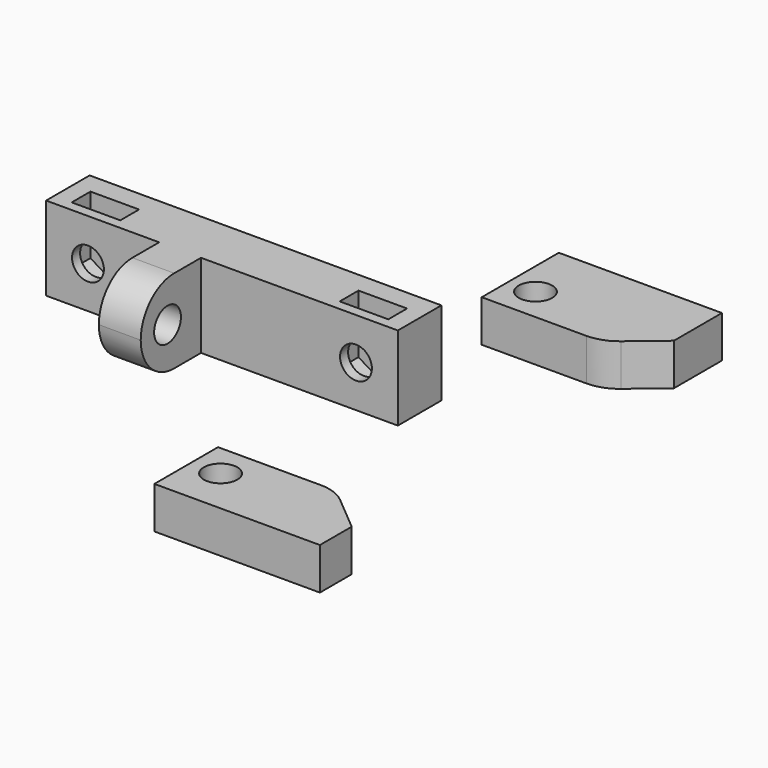
from build123d import *

# Parameters (mm, degrees)
F0_R          = 2
F1_DEPTH      = 5
F2_W          = 5
F2_H          = 9
F3_DEPTH      = 10
F4_R          = 4.99999
F5_R          = 2
F6_DEPTH      = 25
F7_R          = 1.9
F8_DEPTH      = 25
F9_W          = 5.8
F9_H          = 2.8
F10_DEPTH     = 7
F12_DEPTH     = 2.8
F13_TEXT_SIZE = 5.6005794451
F14_DEPTH     = 0.5


# Not quite as in the source:
# - a fillet or chamfer is up to 0.001 mm smaller than in the source, because OpenCascade refuses the exact size
# - Text() gives the source's letters only with a copy of the font that has no kerning and outlines rounded to 1/6400 em; it was checked with that copy


with BuildPart() as f1:
    # F0 (on Top) → F1 (new body)
    with BuildSketch(Plane.XY):
        with BuildLine():
            Line((-19.0093460243, 27.9687746611), (-19.0093460243, 16.4687746611))
            Line((-19.0093460243, 16.4687746611), (-6.5133564216, 16.4687746611))
            ThreePointArc((-6.5133564216, 16.4687746611), (-4.8032557049, 16.7703115571), (-3.2994183731, 17.6385524455))
            Line((-3.2994183731, 17.6385524455), (0.4682703734, 20.8000186831))
            Line((0.4682703734, 20.8000186831), (0.4682703734, 27.9687746611))
            Line((0.4682703734, 27.9687746611), (-19.0093460243, 27.9687746611))
        make_face()
        with Locations((-15.7921736951, 20.4687746611)):
            Circle(F0_R, mode=Mode.SUBTRACT)
    extrude(amount=F1_DEPTH)


with BuildPart() as f1b:
    # F0 (on Top) → F1, piece 2 (new body)
    with BuildSketch(Plane.XY):
        with BuildLine():
            Line((-19.2959401757, -22.5312253389), (-19.2959401757, -32.0312253389))
            Line((-19.2959401757, -32.0312253389), (0.4682703734, -32.0312253389))
            Line((0.4682703734, -32.0312253389), (0.4682703734, -27.2812253389))
            Line((0.4682703734, -27.2812253389), (-3.7984723143, -23.7010031233))
            ThreePointArc((-3.7984723143, -23.7010031233), (-5.3023096461, -22.832762235), (-7.0124103627, -22.5312253389))
            Line((-7.0124103627, -22.5312253389), (-19.2959401757, -22.5312253389))
        make_face()
        with Locations((-15.7921736951, -26.5312253389)):
            Circle(F0_R, mode=Mode.SUBTRACT)
    extrude(amount=F1_DEPTH)


with BuildPart() as f3:
    # F2 (on Top) → F3 (new body)
    with BuildSketch(Plane.XY):
        Polygon((-14.9205976129, 5.3368465819), (-56.9205976129, 5.3368465819), (-56.9205976129, -1.1631534181), (-43.4205976129, -1.1631534181), (-38.4205976129, -1.1631534181), (-14.9205976129, -1.1631534181), align=None)
        with Locations((-40.9205976129, -5.6631534181)):
            Rectangle(F2_W, F2_H)
    extrude(amount=F3_DEPTH)

    # F4 (radius 5 in the source; OpenCascade refuses exactly that, so slightly less here)
    f4_edges = [f3.edges().sort_by_distance(p)[0] for p in [
        (-40.920598, -10.163153, 10),
        (-40.920598, -10.163153, 0),
    ]]
    fillet(f4_edges, radius=F4_R)

    # F5 (on face) → F6 (cut)
    with BuildSketch(Plane(origin=(-43.4205976129, 0, 0), x_dir=(0, -1, 0), z_dir=(-1, 0, 0))):
        with Locations((6.1631534181, 5)):
            Circle(F5_R)
    extrude(amount=-F6_DEPTH, mode=Mode.SUBTRACT)

    # F7 (on face) → F8 (cut)
    with BuildSketch(Plane.XZ.offset(1.1631534181)):
        with Locations((-51.9205976129, 5)):
            Circle(F7_R)
        with Locations((-19.9205976129, 5)):
            Circle(F7_R)
    extrude(amount=-F8_DEPTH, mode=Mode.SUBTRACT)

    # F9 (on face) → F10 (cut)
    with BuildSketch(Plane.XY.offset(10)):
        with Locations((-19.9205976129, 1.4368465819)):
            Rectangle(F9_W, F9_H)
        with Locations((-51.9205976129, 1.4368465819)):
            Rectangle(F9_W, F9_H)
    extrude(amount=-F10_DEPTH, mode=Mode.SUBTRACT)

    # F11 (on face) → F12 (cut)
    with BuildSketch(Plane.XZ.offset(-2.8368465819)):
        Polygon((-49.0205976129, 3), (-54.8205976129, 3), (-51.9205976129, 1.2251760651), align=None)
        Polygon((-17.0205976129, 3), (-22.8205976129, 3), (-19.9205976129, 1.2251760651), align=None)
    extrude(amount=F12_DEPTH, mode=Mode.SUBTRACT)

    # F13 (on face) → F14 (cut)
    with BuildSketch(Plane(origin=(0, 0, 0), x_dir=(1, 0, 0), z_dir=(0, 0, -1))):
        with Locations((-56.2009140849, -4.0324172005)):
            Text('X16 v0.1 RC1.0', F13_TEXT_SIZE, font='Open Sans', text_align=(TextAlign.LEFT, TextAlign.BOTTOM))
    extrude(amount=-F14_DEPTH, mode=Mode.SUBTRACT)


solid = Compound([f1.part, f1b.part, f3.part])
